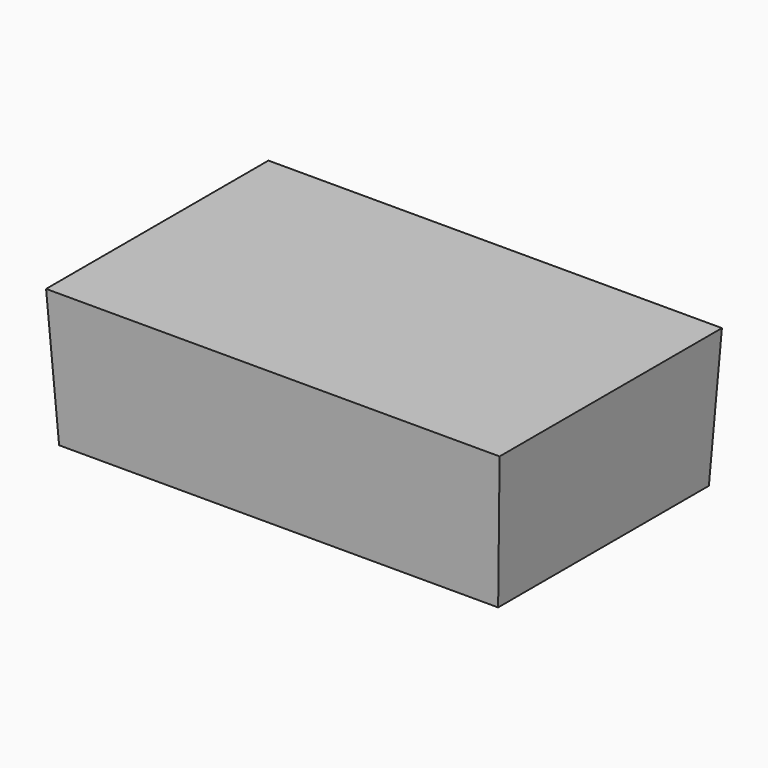
from build123d import *

# Parameters (mm, degrees)
F1_W     = 31.75
F1_H     = 19.05
F2_DEPTH = 10
F2_TAPER = -3


with BuildPart() as f2:
    # F1 (on Top) → F2 (new body)
    with BuildSketch(Plane.XY):
        with Locations((-15.875, 9.525)):
            Rectangle(F1_W, F1_H)
    extrude(amount=F2_DEPTH, taper=F2_TAPER)


solid = f2.part
